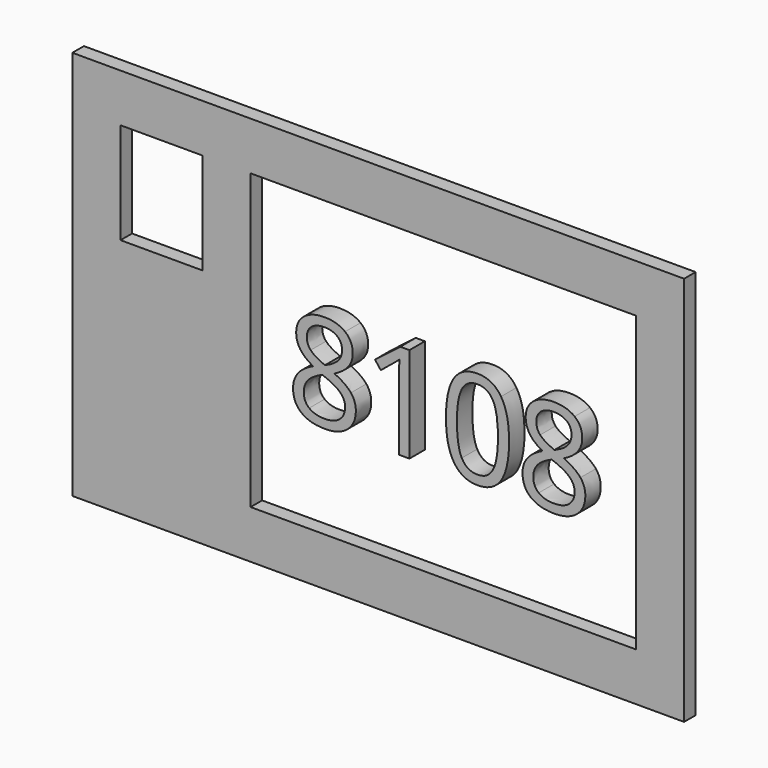
from build123d import *

# Parameters (mm, degrees)
F0_W     = 107.95
F0_H     = 63.5
F1_DEPTH = 19.05
F2_DEPTH = 25.4
F3_DEPTH = 25.4
F4_DEPTH = 19.05


# Not quite as in the source:
# - a feature names something its author has since deleted; it is built from what else it names


with BuildPart() as f1:
    # F0 (on Front) → F1 (new body)
    with BuildSketch(Plane.XZ):
        Polygon((-339.725, 193.675), (-403.225, 257.175), (-403.225, -257.175), (-339.725, -193.675), (-339.725, -130.175), (-339.725, -66.675), (-339.725, -3.175), (-339.725, 60.325), align=None)
        Polygon((-168.275, 193.675), (339.725, 193.675), (403.225, 257.175), (-403.225, 257.175), (-339.725, 193.675), (-231.775, 193.675), align=None)
        Polygon((403.225, 257.175), (339.725, 193.675), (339.725, -193.675), (403.225, -257.175), align=None)
        Polygon((403.225, -257.175), (339.725, -193.675), (-168.275, -193.675), (-231.775, -193.675), (-339.725, -193.675), (-403.225, -257.175), align=None)
        Polygon((-168.275, -193.675), (-168.275, 193.675), (-231.775, 193.675), (-231.775, 60.325), (-231.775, -3.175), (-231.775, -66.675), (-231.775, -130.175), (-231.775, -193.675), align=None)
        with Locations((-285.75, -161.925)):
            Rectangle(F0_W, F0_H)
        with Locations((-285.75, -34.925)):
            Rectangle(F0_W, F0_H)
        with Locations((-285.75, 28.575)):
            Rectangle(F0_W, F0_H)
    extrude(amount=F1_DEPTH)

    # F0 (on Front) → F4 (join)
    with BuildSketch(Plane.XZ):
        with Locations((-285.75, -98.425)):
            Rectangle(F0_W, F0_H)
    extrude(amount=F4_DEPTH)


with BuildPart() as f2:
    # F0 (on Front) → F2 (new body)
    with BuildSketch(Plane.XZ):
        with BuildLine():
            add(Edge.make_bspline(
                [(-65.8594583948, 62.6082563914), (-48.6339809642, 62.6082563914), (-38.5605217628, 54.6018544816)],
                knots=[0, 0, 0, 1, 1, 1], degree=2))
            add(Edge.make_bspline(
                [(-92.9516892975, 54.4778310441), (-82.8368889503, 62.6082563914), (-65.8594583948, 62.6082563914)],
                knots=[0, 0, 0, 1, 1, 1], degree=2))
            add(Edge.make_bspline(
                [(-103.0664896448, 32.6497060441), (-103.0664896448, 46.3474056969), (-92.9516892975, 54.4778310441)],
                knots=[0, 0, 0, 1, 1, 1], degree=2))
            add(Edge.make_bspline(
                [(-97.8988464156, 15.2037425025), (-103.0664896448, 23.003438683), (-103.0664896448, 32.6497060441)],
                knots=[0, 0, 0, 1, 1, 1], degree=2))
            add(Edge.make_bspline(
                [(-80.8525139503, 0.7067806969), (-92.7312031864, 7.4040463219), (-97.8988464156, 15.2037425025)],
                knots=[0, 0, 0, 1, 1, 1], degree=2))
            add(Edge.make_bspline(
                [(-107.2006042281, -32.9724727753), (-107.2006042281, -11.3648338864), (-80.8525139503, 0.7067806969)],
                knots=[0, 0, 0, 1, 1, 1], degree=2))
            add(Edge.make_bspline(
                [(-96.3416632559, -58.0114267684), (-107.2006042281, -49.178201942), (-107.2006042281, -32.9724727753)],
                knots=[0, 0, 0, 1, 1, 1], degree=2))
            add(Edge.make_bspline(
                [(-65.3358038809, -66.8446515948), (-85.4827222837, -66.8446515948), (-96.3416632559, -58.0114267684)],
                knots=[0, 0, 0, 1, 1, 1], degree=2))
            add(Edge.make_bspline(
                [(-35.3772535337, -57.4877722545), (-46.3188767975, -66.8446515948), (-65.3358038809, -66.8446515948)],
                knots=[0, 0, 0, 1, 1, 1], degree=2))
            add(Edge.make_bspline(
                [(-24.4356302698, -32.4763790253), (-24.4356302698, -48.1308929142), (-35.3772535337, -57.4877722545)],
                knots=[0, 0, 0, 1, 1, 1], degree=2))
            add(Edge.make_bspline(
                [(-30.8986294017, -13.8177418725), (-24.4356302698, -21.8654849281), (-24.4356302698, -32.4763790253)],
                knots=[0, 0, 0, 1, 1, 1], degree=2))
            add(Edge.make_bspline(
                [(-52.6854132559, 1.5611643775), (-37.3616285337, -5.769998817), (-30.8986294017, -13.8177418725)],
                knots=[0, 0, 0, 1, 1, 1], degree=2))
            add(Edge.make_bspline(
                [(-34.2472622142, 15.5069109052), (-40.007461867, 7.8450185441), (-52.6854132559, 1.5611643775)],
                knots=[0, 0, 0, 1, 1, 1], degree=2))
            add(Edge.make_bspline(
                [(-28.4870625614, 32.4843414608), (-28.4870625614, 23.1688032664), (-34.2472622142, 15.5069109052)],
                knots=[0, 0, 0, 1, 1, 1], degree=2))
            add(Edge.make_bspline(
                [(-38.5605217628, 54.6018544816), (-28.4870625614, 46.5954525719), (-28.4870625614, 32.4843414608)],
                knots=[0, 0, 0, 1, 1, 1], degree=2))
        make_face()
        with BuildLine():
            add(Edge.make_bspline(
                [(-93.0619323531, -33.3307627059), (-93.0619323531, -43.6660491642), (-85.88235336, -49.4400291989)],
                knots=[0, 0, 0, 1, 1, 1], degree=2))
            add(Edge.make_bspline(
                [(-87.3017327003, -17.3455196503), (-93.0619323531, -24.0152245114), (-93.0619323531, -33.3307627059)],
                knots=[0, 0, 0, 1, 1, 1], degree=2))
            add(Edge.make_bspline(
                [(-68.6982170753, -5.1636620114), (-81.5415330475, -10.6758147892), (-87.3017327003, -17.3455196503)],
                knots=[0, 0, 0, 1, 1, 1], degree=2))
            add(Edge.make_bspline(
                [(-45.2715677698, -17.7864918725), (-51.9963941587, -11.2821515948), (-68.6982170753, -5.1636620114)],
                knots=[0, 0, 0, 1, 1, 1], degree=2))
            add(Edge.make_bspline(
                [(-38.5467413809, -32.6417436086), (-38.5467413809, -24.2908321503), (-45.2715677698, -17.7864918725)],
                knots=[0, 0, 0, 1, 1, 1], degree=2))
            add(Edge.make_bspline(
                [(-45.69875961, -49.178201942), (-38.5467413809, -43.1423946503), (-38.5467413809, -32.6417436086)],
                knots=[0, 0, 0, 1, 1, 1], degree=2))
            add(Edge.make_bspline(
                [(-65.6940938114, -55.2140092336), (-52.8507778392, -55.2140092336), (-45.69875961, -49.178201942)],
                knots=[0, 0, 0, 1, 1, 1], degree=2))
            add(Edge.make_bspline(
                [(-85.88235336, -49.4400291989), (-78.702774367, -55.2140092336), (-65.6940938114, -55.2140092336)],
                knots=[0, 0, 0, 1, 1, 1], degree=2))
        make_face(mode=Mode.SUBTRACT)
        with BuildLine():
            add(Edge.make_bspline(
                [(-66.0248229781, 51.0051747941), (-76.8010816587, 51.0051747941), (-82.919571242, 45.837531565)],
                knots=[0, 0, 0, 1, 1, 1], degree=2))
            add(Edge.make_bspline(
                [(-48.8406866934, 45.8788727108), (-55.0831997142, 51.0051747941), (-66.0248229781, 51.0051747941)],
                knots=[0, 0, 0, 1, 1, 1], degree=2))
            add(Edge.make_bspline(
                [(-42.5981736725, 32.0433692386), (-42.5981736725, 40.7525706275), (-48.8406866934, 45.8788727108)],
                knots=[0, 0, 0, 1, 1, 1], degree=2))
            add(Edge.make_bspline(
                [(-47.7244757559, 18.1803050025), (-42.5981736725, 24.1334300025), (-42.5981736725, 32.0433692386)],
                knots=[0, 0, 0, 1, 1, 1], degree=2))
            add(Edge.make_bspline(
                [(-65.1704392975, 7.0733171552), (-52.8507778392, 12.2271800025), (-47.7244757559, 18.1803050025)],
                knots=[0, 0, 0, 1, 1, 1], degree=2))
            add(Edge.make_bspline(
                [(-83.9530998878, 18.4421322594), (-78.8681389503, 12.7508345164), (-65.1704392975, 7.0733171552)],
                knots=[0, 0, 0, 1, 1, 1], degree=2))
            add(Edge.make_bspline(
                [(-89.0380608253, 32.0433692386), (-89.0380608253, 24.1334300025), (-83.9530998878, 18.4421322594)],
                knots=[0, 0, 0, 1, 1, 1], degree=2))
            add(Edge.make_bspline(
                [(-82.919571242, 45.837531565), (-89.0380608253, 40.6698883358), (-89.0380608253, 32.0433692386)],
                knots=[0, 0, 0, 1, 1, 1], degree=2))
        make_face(mode=Mode.SUBTRACT)
    extrude(amount=F2_DEPTH)


with BuildPart() as f3:
    # F0 (on Front) → F3 (new body)
    with BuildSketch(Plane.XZ):
        with BuildLine():
            Line((32.3119825775, -65.1083234698), (46.2577291052, -65.1083234698))
            Line((46.2577291052, -65.1083234698), (46.2577291052, 60.8168067386))
            Line((46.2577291052, 60.8168067386), (34.2136752858, 60.8168067386))
            Line((34.2136752858, 60.8168067386), (0.8927117441, 35.0474925025))
            Line((0.8927117441, 35.0474925025), (8.4719218136, 25.235860558))
            add(Edge.make_bspline(
                [(28.963349765, 42.0341461483), (26.717147508, 40.0635515302), (8.4719218136, 25.235860558)],
                knots=[0, 0, 0, 1, 1, 1], degree=2))
            add(Edge.make_bspline(
                [(33.0010016747, 45.823751183), (31.2095520219, 44.0047407664), (28.963349765, 42.0341461483)],
                knots=[0, 0, 0, 1, 1, 1], degree=2))
            add(Edge.make_bspline(
                [(32.3119825775, 24.6295237525), (32.3119825775, 35.8467546552), (33.0010016747, 45.823751183)],
                knots=[0, 0, 0, 1, 1, 1], degree=2))
            Line((32.3119825775, 24.6295237525), (32.3119825775, -65.1083234698))
        make_face()
        with BuildLine():
            add(Edge.make_bspline(
                [(177.6123297997, -1.9666134003), (177.6123297997, -34.6261186086), (167.3183844872, -50.7353851017)],
                knots=[0, 0, 0, 1, 1, 1], degree=2))
            add(Edge.make_bspline(
                [(166.9738749386, 46.1682607316), (177.6123297997, 29.5353397247), (177.6123297997, -1.9666134003)],
                knots=[0, 0, 0, 1, 1, 1], degree=2))
            add(Edge.make_bspline(
                [(135.8302117441, 62.8011817386), (156.3354200775, 62.8011817386), (166.9738749386, 46.1682607316)],
                knots=[0, 0, 0, 1, 1, 1], degree=2))
            add(Edge.make_bspline(
                [(104.5763054941, 46.8572798289), (114.8289096608, 62.8011817386), (135.8302117441, 62.8011817386)],
                knots=[0, 0, 0, 1, 1, 1], degree=2))
            add(Edge.make_bspline(
                [(94.3237013275, -1.9666134003), (94.3237013275, 30.9133779191), (104.5763054941, 46.8572798289)],
                knots=[0, 0, 0, 1, 1, 1], degree=2))
            add(Edge.make_bspline(
                [(104.9208150427, -50.3495344073), (94.3237013275, -33.8544172198), (94.3237013275, -1.9666134003)],
                knots=[0, 0, 0, 1, 1, 1], degree=2))
            add(Edge.make_bspline(
                [(135.8302117441, -66.8446515948), (115.517928758, -66.8446515948), (104.9208150427, -50.3495344073)],
                knots=[0, 0, 0, 1, 1, 1], degree=2))
            add(Edge.make_bspline(
                [(167.3183844872, -50.7353851017), (157.0244391747, -66.8446515948), (135.8302117441, -66.8446515948)],
                knots=[0, 0, 0, 1, 1, 1], degree=2))
        make_face()
        with BuildLine():
            add(Edge.make_bspline(
                [(108.7931023691, -1.9666134003), (108.7931023691, -29.4446949975), (115.2561015011, -41.984842567)],
                knots=[0, 0, 0, 1, 1, 1], degree=2))
            add(Edge.make_bspline(
                [(115.2561015011, 37.9551530927), (108.7931023691, 25.5114681969), (108.7931023691, -1.9666134003)],
                knots=[0, 0, 0, 1, 1, 1], degree=2))
            add(Edge.make_bspline(
                [(135.8302117441, 50.3988379886), (121.719100633, 50.3988379886), (115.2561015011, 37.9551530927)],
                knots=[0, 0, 0, 1, 1, 1], degree=2))
            add(Edge.make_bspline(
                [(156.5421258066, 37.7760081275), (150.1342482025, 50.3988379886), (135.8302117441, 50.3988379886)],
                knots=[0, 0, 0, 1, 1, 1], degree=2))
            add(Edge.make_bspline(
                [(162.9500034108, -1.9666134003), (162.9500034108, 25.1531782664), (156.5421258066, 37.7760081275)],
                knots=[0, 0, 0, 1, 1, 1], degree=2))
            add(Edge.make_bspline(
                [(156.5421258066, -41.8194779836), (162.9500034108, -29.1139658309), (162.9500034108, -1.9666134003)],
                knots=[0, 0, 0, 1, 1, 1], degree=2))
            add(Edge.make_bspline(
                [(135.8302117441, -54.5249901364), (150.1342482025, -54.5249901364), (156.5421258066, -41.8194779836)],
                knots=[0, 0, 0, 1, 1, 1], degree=2))
            add(Edge.make_bspline(
                [(115.2561015011, -41.984842567), (121.719100633, -54.5249901364), (135.8302117441, -54.5249901364)],
                knots=[0, 0, 0, 1, 1, 1], degree=2))
        make_face(mode=Mode.SUBTRACT)
        with BuildLine():
            add(Edge.make_bspline(
                [(236.6750468136, 62.6082563914), (253.9005242441, 62.6082563914), (263.9739834455, 54.6018544816)],
                knots=[0, 0, 0, 1, 1, 1], degree=2))
            add(Edge.make_bspline(
                [(209.5828159108, 54.4778310441), (219.697616258, 62.6082563914), (236.6750468136, 62.6082563914)],
                knots=[0, 0, 0, 1, 1, 1], degree=2))
            add(Edge.make_bspline(
                [(199.4680155636, 32.6497060441), (199.4680155636, 46.3474056969), (209.5828159108, 54.4778310441)],
                knots=[0, 0, 0, 1, 1, 1], degree=2))
            add(Edge.make_bspline(
                [(204.6356587927, 15.2037425025), (199.4680155636, 23.003438683), (199.4680155636, 32.6497060441)],
                knots=[0, 0, 0, 1, 1, 1], degree=2))
            add(Edge.make_bspline(
                [(221.681991258, 0.7067806969), (209.8033020219, 7.4040463219), (204.6356587927, 15.2037425025)],
                knots=[0, 0, 0, 1, 1, 1], degree=2))
            add(Edge.make_bspline(
                [(195.3339009802, -32.9724727753), (195.3339009802, -11.3648338864), (221.681991258, 0.7067806969)],
                knots=[0, 0, 0, 1, 1, 1], degree=2))
            add(Edge.make_bspline(
                [(206.1928419525, -58.0114267684), (195.3339009802, -49.178201942), (195.3339009802, -32.9724727753)],
                knots=[0, 0, 0, 1, 1, 1], degree=2))
            add(Edge.make_bspline(
                [(237.1987013275, -66.8446515948), (217.0517829247, -66.8446515948), (206.1928419525, -58.0114267684)],
                knots=[0, 0, 0, 1, 1, 1], degree=2))
            add(Edge.make_bspline(
                [(267.1572516747, -57.4877722545), (256.2156284108, -66.8446515948), (237.1987013275, -66.8446515948)],
                knots=[0, 0, 0, 1, 1, 1], degree=2))
            add(Edge.make_bspline(
                [(278.0988749386, -32.4763790253), (278.0988749386, -48.1308929142), (267.1572516747, -57.4877722545)],
                knots=[0, 0, 0, 1, 1, 1], degree=2))
            add(Edge.make_bspline(
                [(271.6358758066, -13.8177418725), (278.0988749386, -21.8654849281), (278.0988749386, -32.4763790253)],
                knots=[0, 0, 0, 1, 1, 1], degree=2))
            add(Edge.make_bspline(
                [(249.8490919525, 1.5611643775), (265.1728766747, -5.769998817), (271.6358758066, -13.8177418725)],
                knots=[0, 0, 0, 1, 1, 1], degree=2))
            add(Edge.make_bspline(
                [(268.2872429941, 15.5069109052), (262.5270433413, 7.8450185441), (249.8490919525, 1.5611643775)],
                knots=[0, 0, 0, 1, 1, 1], degree=2))
            add(Edge.make_bspline(
                [(274.0474426469, 32.4843414608), (274.0474426469, 23.1688032664), (268.2872429941, 15.5069109052)],
                knots=[0, 0, 0, 1, 1, 1], degree=2))
            add(Edge.make_bspline(
                [(263.9739834455, 54.6018544816), (274.0474426469, 46.5954525719), (274.0474426469, 32.4843414608)],
                knots=[0, 0, 0, 1, 1, 1], degree=2))
        make_face()
        with BuildLine():
            add(Edge.make_bspline(
                [(209.4725728552, -33.3307627059), (209.4725728552, -43.6660491642), (216.6521518483, -49.4400291989)],
                knots=[0, 0, 0, 1, 1, 1], degree=2))
            add(Edge.make_bspline(
                [(215.232772508, -17.3455196503), (209.4725728552, -24.0152245114), (209.4725728552, -33.3307627059)],
                knots=[0, 0, 0, 1, 1, 1], degree=2))
            add(Edge.make_bspline(
                [(233.836288133, -5.1636620114), (220.9929721608, -10.6758147892), (215.232772508, -17.3455196503)],
                knots=[0, 0, 0, 1, 1, 1], degree=2))
            add(Edge.make_bspline(
                [(257.2629374386, -17.7864918725), (250.5381110497, -11.2821515948), (233.836288133, -5.1636620114)],
                knots=[0, 0, 0, 1, 1, 1], degree=2))
            add(Edge.make_bspline(
                [(263.9877638275, -32.6417436086), (263.9877638275, -24.2908321503), (257.2629374386, -17.7864918725)],
                knots=[0, 0, 0, 1, 1, 1], degree=2))
            add(Edge.make_bspline(
                [(256.8357455983, -49.178201942), (263.9877638275, -43.1423946503), (263.9877638275, -32.6417436086)],
                knots=[0, 0, 0, 1, 1, 1], degree=2))
            add(Edge.make_bspline(
                [(236.8404113969, -55.2140092336), (249.6837273691, -55.2140092336), (256.8357455983, -49.178201942)],
                knots=[0, 0, 0, 1, 1, 1], degree=2))
            add(Edge.make_bspline(
                [(216.6521518483, -49.4400291989), (223.8317308413, -55.2140092336), (236.8404113969, -55.2140092336)],
                knots=[0, 0, 0, 1, 1, 1], degree=2))
        make_face(mode=Mode.SUBTRACT)
        with BuildLine():
            add(Edge.make_bspline(
                [(236.5096822302, 51.0051747941), (225.7334235497, 51.0051747941), (219.6149339663, 45.837531565)],
                knots=[0, 0, 0, 1, 1, 1], degree=2))
            add(Edge.make_bspline(
                [(253.693818515, 45.8788727108), (247.4513054941, 51.0051747941), (236.5096822302, 51.0051747941)],
                knots=[0, 0, 0, 1, 1, 1], degree=2))
            add(Edge.make_bspline(
                [(259.9363315358, 32.0433692386), (259.9363315358, 40.7525706275), (253.693818515, 45.8788727108)],
                knots=[0, 0, 0, 1, 1, 1], degree=2))
            add(Edge.make_bspline(
                [(254.8100294525, 18.1803050025), (259.9363315358, 24.1334300025), (259.9363315358, 32.0433692386)],
                knots=[0, 0, 0, 1, 1, 1], degree=2))
            add(Edge.make_bspline(
                [(237.3640659108, 7.0733171552), (249.6837273691, 12.2271800025), (254.8100294525, 18.1803050025)],
                knots=[0, 0, 0, 1, 1, 1], degree=2))
            add(Edge.make_bspline(
                [(218.5814053205, 18.4421322594), (223.666366258, 12.7508345164), (237.3640659108, 7.0733171552)],
                knots=[0, 0, 0, 1, 1, 1], degree=2))
            add(Edge.make_bspline(
                [(213.496444383, 32.0433692386), (213.496444383, 24.1334300025), (218.5814053205, 18.4421322594)],
                knots=[0, 0, 0, 1, 1, 1], degree=2))
            add(Edge.make_bspline(
                [(219.6149339663, 45.837531565), (213.496444383, 40.6698883358), (213.496444383, 32.0433692386)],
                knots=[0, 0, 0, 1, 1, 1], degree=2))
        make_face(mode=Mode.SUBTRACT)
    extrude(amount=F3_DEPTH)


solid = Compound([f1.part, f2.part, f3.part])
